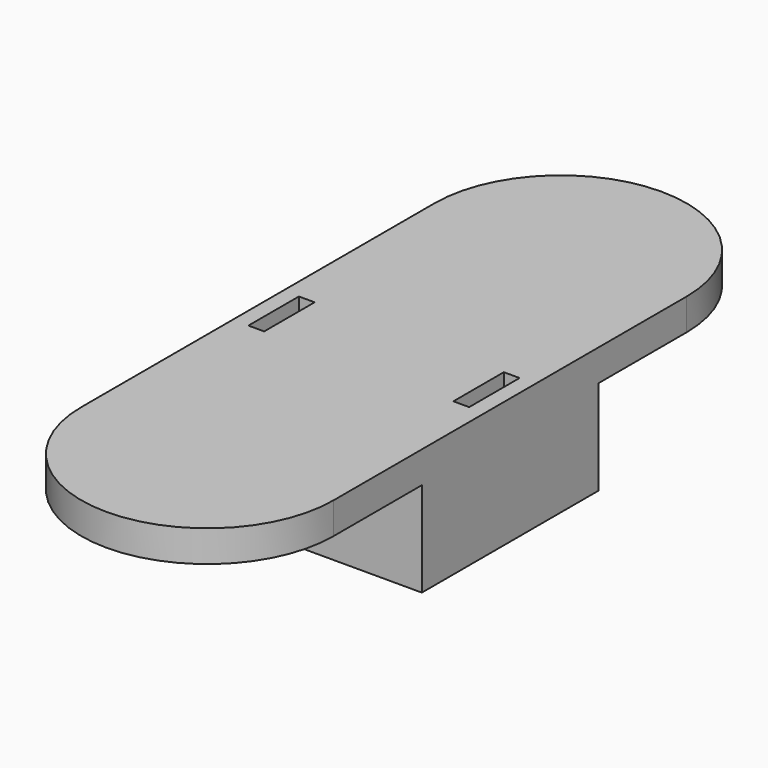
from build123d import *

# Parameters (mm, degrees)
F1_DEPTH = 12.7
F2_W     = 101.6
F2_H     = 88.9
F3_DEPTH = 38.1
F5_D     = 25.4
F5_DEPTH = 76.2
F5_TIP   = 7.6309298617
F6_W     = 6.35
F6_H     = 25.4
F7_DEPTH = 6.35
F8_W     = 88.9
F8_H     = 27.94
F9_DEPTH = 6.35


with BuildPart() as f1:
    # F0 (on Top) → F1 (new body)
    with BuildSketch(Plane.XY):
        with BuildLine():
            Line((-50.8, 88.9), (-50.8, -88.9))
            ThreePointArc((-50.8, -88.9), (0, -139.7), (50.8, -88.9))
            Line((50.8, -88.9), (50.8, 88.9))
            ThreePointArc((50.8, 88.9), (0, 139.7), (-50.8, 88.9))
        make_face()
    extrude(amount=F1_DEPTH)

    # F2 (on face) → F3 (join)
    with BuildSketch(Plane(origin=(0, 0, 0), x_dir=(1, 0, 0), z_dir=(0, 0, -1))):
        Rectangle(F2_W, F2_H)
    extrude(amount=F3_DEPTH)

    # F5
    with Locations(Plane(origin=(-50.8, 0, 0), x_dir=(0, -1, 0), z_dir=(-1, 0, 0))):
        with Locations((0, -19.05)):
            Hole(F5_D / 2, depth=F5_DEPTH)
            with Locations((0, 0, -(F5_DEPTH + F5_TIP / 2))):  # 118° drill point
                Cone(0, F5_D / 2, F5_TIP, mode=Mode.SUBTRACT)

    # F6 (on face) → F7 (cut)
    with BuildSketch(Plane.XY.offset(12.7)):
        with Locations((-41.275, 0)):
            Rectangle(F6_W, F6_H)
        with Locations((41.275, 0)):
            Rectangle(F6_W, F6_H)
    extrude(amount=-F7_DEPTH, mode=Mode.SUBTRACT)

    # F8 (on face) → F9 (cut)
    with BuildSketch(Plane(origin=(0, 0, 0), x_dir=(1, 0, 0), z_dir=(0, 0, -1))):
        Rectangle(F8_W, F8_H)
    extrude(amount=-F9_DEPTH, mode=Mode.SUBTRACT)


solid = f1.part
